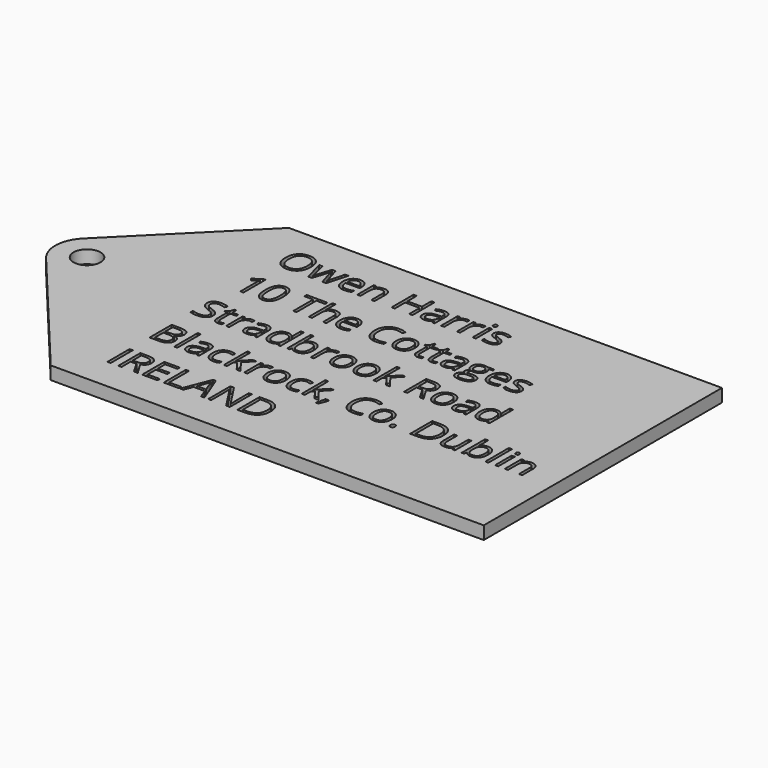
from build123d import *

# Parameters (mm, degrees)
F0_R         = 2.5
F0_W         = 80
F0_H         = 55
F1_DEPTH     = 2.4
F2_TEXT_SIZE = 7.1451355662
F3_DEPTH     = 1.2


# Not quite as in the source:
# - Text() gives the source's letters only with a copy of the font that has no kerning and outlines rounded to 1/6400 em; it was checked with that copy


with BuildPart() as f1:
    # F0 (on Top) → F1 (new body)
    with BuildSketch(Plane.XY):
        with BuildLine():
            Line((-28.865801543, -30), (-28.865801543, 25))
            Line((-28.865801543, 25), (-49.9913599641, 3.8744415789))
            ThreePointArc((-49.9913599641, 3.8744415789), (-51.7425559211, -0.0963125811), (-50.3580469545, -4.2093055062))
            Line((-50.3580469545, -4.2093055062), (-28.865801543, -30))
        make_face()
        with Locations((-45.865801543, -0.3681991082)):
            Circle(F0_R, mode=Mode.SUBTRACT)
        with Locations((11.134198457, -2.5)):
            Rectangle(F0_W, F0_H)
    extrude(amount=F1_DEPTH)

    # F2 (on face) → F3 (cut)
    with BuildSketch(Plane.XY.offset(2.4)):
        with Locations((-23.865801543, 14.8555023923)):
            Text('Owen Harris', F2_TEXT_SIZE, font='Open Sans', text_align=(TextAlign.LEFT, TextAlign.BOTTOM))
        with Locations((-23.865801543, 5.1381180223)):
            Text('10 The Cottages', F2_TEXT_SIZE, font='Open Sans', text_align=(TextAlign.LEFT, TextAlign.BOTTOM))
        with Locations((-23.865801543, -4.5792663477)):
            Text('Stradbrook Road', F2_TEXT_SIZE, font='Open Sans', text_align=(TextAlign.LEFT, TextAlign.BOTTOM))
        with Locations((-23.865801543, -14.2966507177)):
            Text('Blackrock, Co. Dublin', F2_TEXT_SIZE, font='Open Sans', text_align=(TextAlign.LEFT, TextAlign.BOTTOM))
        with Locations((-23.865801543, -24.0140350877)):
            Text('IRELAND', F2_TEXT_SIZE, font='Open Sans', text_align=(TextAlign.LEFT, TextAlign.BOTTOM))
    extrude(amount=-F3_DEPTH, mode=Mode.SUBTRACT)


solid = f1.part
